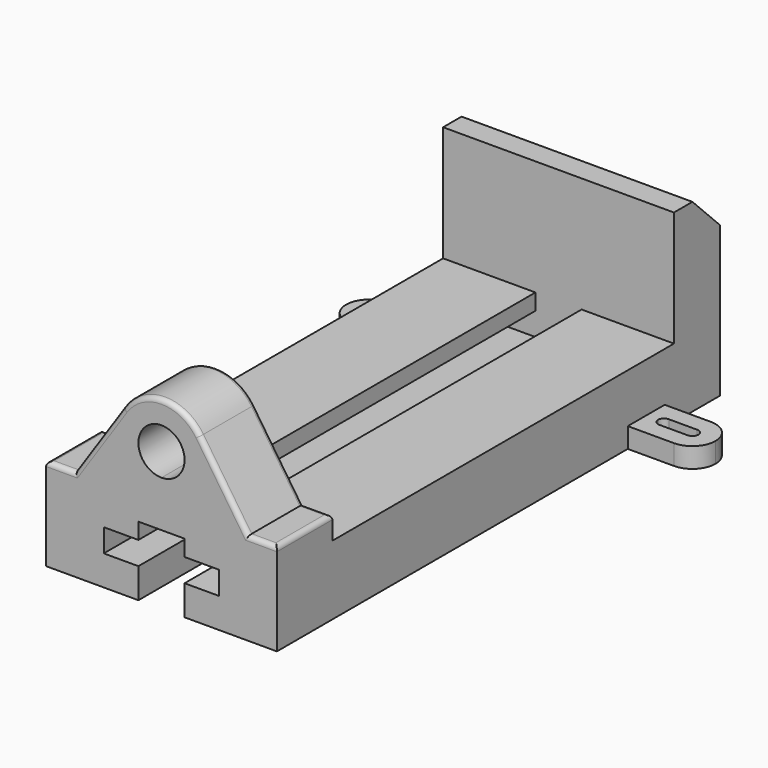
from build123d import *

# Parameters (mm, degrees)
F1_DEPTH  = 38.1
F3_DEPTH  = 273.05
F4_W      = 25.4
F4_H      = 38.1
F4_W_2    = 50.8
F5_DEPTH  = 12.7
F7_DEPTH  = 38.1
F8_R      = 2.54
F10_DEPTH = 11.049
F11_DEPTH = 11.049
F12_DEPTH = 63.5
F13_SIZE  = 19.05


with BuildPart() as f1:
    # F0 (on Top) → F1 (new body)
    with BuildSketch(Plane.XY):
        Polygon((-63.5, -152.4), (63.5, -152.4), (63.5, 88.9), (63.5, 101.6), (63.5, 114.3), (63.5, 152.4), (-63.5, 152.4), (-63.5, 114.3), (-63.5, 101.6), (-63.5, 88.9), align=None)
    extrude(amount=F1_DEPTH)

    # F2 (on face) → F3 (cut)
    with BuildSketch(Plane.XZ.offset(152.4)):
        Polygon((-12.7, 0), (0, 0), (12.7, 0), (12.7, 16.51), (31.75, 16.51), (31.75, 29.21), (12.7, 29.21), (12.7, 38.1), (-12.7, 38.1), (-12.7, 29.21), (-31.75, 29.21), (-31.75, 16.51), (-12.7, 16.51), align=None)
    extrude(amount=-F3_DEPTH, mode=Mode.SUBTRACT)

    # F4 (on face) → F5 (join)
    with BuildSketch(Plane.XY.offset(38.1)):
        with Locations((0, -133.35)):
            Rectangle(F4_W, F4_H)
        with Locations((-38.1, -133.35)):
            Rectangle(F4_W_2, F4_H)
        with Locations((38.1, -133.35)):
            Rectangle(F4_W_2, F4_H)
    extrude(amount=F5_DEPTH)

    # F6 (on face) → F7 (join)
    with BuildSketch(Plane.XZ.offset(152.4)):
        with BuildLine():
            Line((-47.625, 50.8), (0, 50.8))
            Line((0, 50.8), (47.625, 50.8))
            Line((47.625, 50.8), (21.0934256055, 90.3501730104))
            ThreePointArc((21.0934256055, 90.3501730104), (0, 101.6), (-21.0934256055, 90.3501730104))
            Line((-21.0934256055, 90.3501730104), (-47.625, 50.8))
        make_face()
        with BuildLine():
            ThreePointArc((12.7, 76.2), (8.9802561211, 67.2197438789), (0, 63.5))
            ThreePointArc((0, 63.5), (-8.9802561211, 85.1802561211), (12.7, 76.2))
        make_face(mode=Mode.SUBTRACT)
    extrude(amount=-F7_DEPTH)

    # F8
    f8_edges = [f1.edges().sort_by_distance(p)[0] for p in [
        (-55.5625, -152.4, 50.8),
        (55.5625, -152.4, 50.8),
        (34.359213, -152.4, 70.575087),
        (63.5, -133.35, 50.8),
        (-55.5625, -114.3, 50.8),
        (55.5625, -114.3, 50.8),
        (34.359213, -114.3, 70.575087),
        (0, -152.4, 101.6),
        (0, -114.3, 101.6),
        (-34.359213, -152.4, 70.575087),
        (-34.359213, -114.3, 70.575087),
        (-63.5, -133.35, 50.8),
    ]]
    fillet(f8_edges, radius=F8_R)

    # F0 (on Top) → F10 (join)
    with BuildSketch(Plane.XY):
        with BuildLine():
            Line((-88.9, 88.9), (-63.5, 88.9))
            Line((-63.5, 88.9), (-63.5, 101.6))
            Line((-63.5, 101.6), (-69.977, 101.6))
            ThreePointArc((-69.977, 101.6), (-70.9441334085, 99.2651334085), (-73.279, 98.298))
            Line((-73.279, 98.298), (-76.6367705722, 98.298))
            ThreePointArc((-76.6367705722, 98.298), (-81.1748915865, 91.5196875048), (-88.9, 88.9))
        make_face()
        with BuildLine():
            Line((-69.977, 101.6), (-63.5, 101.6))
            Line((-63.5, 101.6), (-63.5, 114.3))
            Line((-63.5, 114.3), (-88.9, 114.3))
            ThreePointArc((-88.9, 114.3), (-81.1748915865, 111.6803124952), (-76.6367705722, 104.902))
            Line((-76.6367705722, 104.902), (-73.279, 104.902))
            ThreePointArc((-73.279, 104.902), (-70.9441334085, 103.9348665915), (-69.977, 101.6))
        make_face()
        with BuildLine():
            Line((-88.9, 98.298), (-88.9, 88.9))
            ThreePointArc((-88.9, 88.9), (-81.1748915865, 91.5196875048), (-76.6367705722, 98.298))
            Line((-76.6367705722, 98.298), (-88.9, 98.298))
        make_face()
        with BuildLine():
            ThreePointArc((-101.6, 101.6), (-97.8802561211, 92.6197438789), (-88.9, 88.9))
            Line((-88.9, 88.9), (-88.9, 98.298))
            ThreePointArc((-88.9, 98.298), (-91.2348665915, 99.2651334085), (-92.202, 101.6))
            Line((-92.202, 101.6), (-101.6, 101.6))
        make_face()
        with BuildLine():
            ThreePointArc((-88.9, 114.3), (-97.8802561211, 110.5802561211), (-101.6, 101.6))
            Line((-101.6, 101.6), (-92.202, 101.6))
            ThreePointArc((-92.202, 101.6), (-91.2348665915, 103.9348665915), (-88.9, 104.902))
            Line((-88.9, 104.902), (-88.9, 114.3))
        make_face()
        with BuildLine():
            ThreePointArc((-76.6367705722, 104.902), (-81.1748915865, 111.6803124952), (-88.9, 114.3))
            Line((-88.9, 114.3), (-88.9, 104.902))
            Line((-88.9, 104.902), (-76.6367705722, 104.902))
        make_face()
    extrude(amount=F10_DEPTH)

    # F0 (on Top) → F11 (join)
    with BuildSketch(Plane.XY):
        with BuildLine():
            Line((63.5, 101.6), (63.5, 88.9))
            Line((63.5, 88.9), (88.9, 88.9))
            ThreePointArc((88.9, 88.9), (81.1748915865, 91.5196875048), (76.6367705722, 98.298))
            Line((76.6367705722, 98.298), (73.279, 98.298))
            ThreePointArc((73.279, 98.298), (70.9441334085, 99.2651334085), (69.977, 101.6))
            Line((69.977, 101.6), (63.5, 101.6))
        make_face()
        with BuildLine():
            ThreePointArc((76.6367705722, 98.298), (81.1748915865, 91.5196875048), (88.9, 88.9))
            Line((88.9, 88.9), (88.9, 98.298))
            Line((88.9, 98.298), (76.6367705722, 98.298))
        make_face()
        with BuildLine():
            Line((92.202, 101.6), (101.6, 101.6))
            ThreePointArc((101.6, 101.6), (97.8802561211, 110.5802561211), (88.9, 114.3))
            Line((88.9, 114.3), (88.9, 104.902))
            ThreePointArc((88.9, 104.902), (91.2348665915, 103.9348665915), (92.202, 101.6))
        make_face()
        with BuildLine():
            Line((88.9, 98.298), (88.9, 88.9))
            ThreePointArc((88.9, 88.9), (97.8802561211, 92.6197438789), (101.6, 101.6))
            Line((101.6, 101.6), (92.202, 101.6))
            ThreePointArc((92.202, 101.6), (91.2348665915, 99.2651334085), (88.9, 98.298))
        make_face()
        with BuildLine():
            Line((88.9, 104.902), (88.9, 114.3))
            ThreePointArc((88.9, 114.3), (81.1748915865, 111.6803124952), (76.6367705722, 104.902))
            Line((76.6367705722, 104.902), (88.9, 104.902))
        make_face()
        with BuildLine():
            Line((63.5, 114.3), (63.5, 101.6))
            Line((63.5, 101.6), (69.977, 101.6))
            ThreePointArc((69.977, 101.6), (70.9441334085, 103.9348665915), (73.279, 104.902))
            Line((73.279, 104.902), (76.6367705722, 104.902))
            ThreePointArc((76.6367705722, 104.902), (81.1748915865, 111.6803124952), (88.9, 114.3))
            Line((88.9, 114.3), (63.5, 114.3))
        make_face()
    extrude(amount=F11_DEPTH)

    # F9 (on face) → F12 (join)
    with BuildSketch(Plane.XY.offset(38.1)):
        Polygon((-63.5, 120.65), (-12.7, 120.65), (12.7, 120.65), (63.5, 120.65), (63.5, 152.4), (-63.5, 152.4), align=None)
    extrude(amount=F12_DEPTH)

    # F13
    f13_edges = [f1.edges().sort_by_distance(p)[0] for p in [
        (0, 152.4, 101.6),
    ]]
    chamfer(f13_edges, length=F13_SIZE)


solid = f1.part
